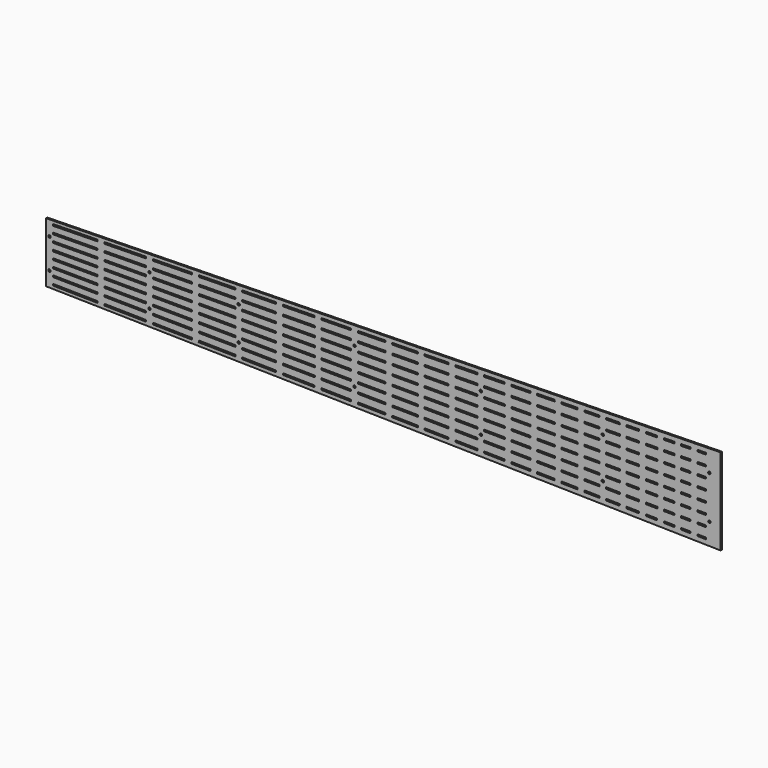
from build123d import *

# Parameters (mm, degrees)
F2_DEPTH = 1.524
F4_DEPTH = 1.525
F5_R     = 1.1303
F6_DEPTH = 985
F7_DEPTH = 1.525


# Not quite as in the source:
# - an extrude ends at something that could not be found from the text; its depth is read off the source's solid


with BuildPart() as f2:
    # F1 (on Front) → F2 (new body)
    with BuildSketch(Plane.XZ):
        Polygon((0, 56.388), (0, 0), (635, -12.446), (635, 68.834), align=None)
    extrude(amount=F2_DEPTH)

    # F0 (on Front) → F4 (cut, through all)
    with BuildSketch(Plane.XZ):
        Polygon((6.3619321188, 4.1792032166), (6.3490994724, 3.4173112799), (6.336266826, 2.6554193432), (48.4507071038, 1.946080269), (48.4635397502, 2.7079722057), (48.4763723966, 3.4698641423), align=None)
        Polygon((54.825471869, 3.3629254222), (54.8126392226, 2.6010334855), (54.7998065761, 1.8391415489), (94.1934291625, 1.175629566), (94.2062618089, 1.9375215027), (94.2190944553, 2.6994134394), align=None)
        Polygon((100.5681939277, 2.5924747193), (100.5553612812, 1.8305827826), (100.5425286348, 1.0686908459), (137.3698960072, 0.4484026382), (137.3827286536, 1.2102945749), (137.3955613, 1.9721865116), align=None)
        Polygon((143.7446607724, 1.8652477915), (143.731828126, 1.1033558548), (143.7189954796, 0.3414639181), (178.1148101324, -0.2378693263), (178.1276427788, 0.5240226104), (178.1404754253, 1.285914547), align=None)
        Polygon((184.4895748976, 1.1789758269), (184.4767422512, 0.4170838902), (184.4639096048, -0.3448080465), (216.5879148808, -0.8858769058), (216.6007475272, -0.1239849691), (216.6135801737, 0.6379069676), align=None)
        Polygon((222.962679646, 0.5309682475), (222.9498469996, -0.2309236892), (222.9370143532, -0.9928156259), (252.8936910333, -1.4973798837), (252.9065236798, -0.7354879471), (252.9193563262, 0.0264039896), align=None)
        Polygon((259.2684557986, -0.0805347305), (259.2556231521, -0.8424266672), (259.2427905057, -1.6043186039), (287.1625236967, -2.0745743538), (287.1753563432, -1.3126824171), (287.1881889896, -0.5507904804), align=None)
        Polygon((293.5372884619, -0.6577292005), (293.5244558155, -1.4196211372), (293.5116231691, -2.1815130739), (319.5075284272, -2.6193655361), (319.5203610736, -1.8574735994), (319.53319372, -1.0955816627), align=None)
        Polygon((325.8822931924, -1.2025203828), (325.869460546, -1.9644123195), (325.8566278996, -2.7263042562), (350.0375033933, -3.1335859326), (350.0503360397, -2.3716939959), (350.0631686861, -1.6098020592), align=None)
        Polygon((356.4122681585, -1.7167407793), (356.3994355121, -2.478632716), (356.3866028657, -3.2405246527), (378.8543389434, -3.6189516959), (378.8671715898, -2.8570597592), (378.8800042362, -2.0951678225), align=None)
        Polygon((385.2291037086, -2.2021065426), (385.2162710622, -2.9639984793), (385.2034384157, -3.725890416), (406.0530176055, -4.0770626292), (406.0658502519, -3.3151706925), (406.0786828983, -2.5532787558), align=None)
        Polygon((412.4277823707, -2.6602174759), (412.4149497243, -3.4221094126), (412.4021170779, -4.1840013493), (431.7259314752, -4.5094749048), (431.7387641216, -3.7475829681), (431.7515967681, -2.9856910314), align=None)
        Polygon((438.1006962404, -3.0926297515), (438.087863594, -3.8545216882), (438.0750309476, -4.6164136249), (455.9577013503, -4.917613802), (455.9705339967, -4.1557218653), (455.9833666431, -3.3938299286), align=None)
        Polygon((462.3324661155, -3.5007686487), (462.3196334691, -4.2626605854), (462.3068008227, -5.0245525221), (478.8294941184, -5.3028464253), (478.8423267648, -4.5409544886), (478.8551594113, -3.7790625519), align=None)
        Polygon((485.2042588836, -3.886001272), (485.1914262372, -4.6478932087), (485.1785935908, -5.4097851454), (500.417295802, -5.6664526173), (500.4301284485, -4.9045606807), (500.4429610949, -4.142668744), align=None)
        Polygon((506.7920605672, -4.2496074641), (506.7792279208, -5.0114994008), (506.7663952744, -5.7733913375), (520.7936385135, -6.0096540461), (520.8064711599, -5.2477621094), (520.8193038064, -4.4858701727), align=None)
        Polygon((527.1684032787, -4.5928088929), (527.1555706323, -5.3547008295), (527.1427379859, -6.1165927662), (540.0258735001, -6.3335851175), (540.0387061465, -5.5716931808), (540.0515387929, -4.8098012441), align=None)
        Polygon((546.4006382653, -4.9167399643), (546.3878056189, -5.6786319009), (546.3749729725, -6.4405238376), (558.1796250539, -6.6393511502), (558.1924577003, -5.8774592135), (558.2052903467, -5.1155672768), align=None)
        Polygon((564.5543898191, -5.2225059969), (564.5415571727, -5.9843979336), (564.5287245263, -6.7462898703), (575.3136096468, -6.9279411133), (575.3264422932, -6.1660491766), (575.3392749396, -5.40415724), align=None)
        Polygon((581.688374412, -5.5110959601), (581.6755417656, -6.2729878968), (581.6627091192, -7.0348798334), (591.4865437508, -7.2003439763), (591.4993763972, -6.4384520396), (591.5122090436, -5.6765601029), align=None)
        Polygon((597.861308516, -5.7834988231), (597.8484758696, -6.5453907597), (597.8356432232, -7.3072826964), (606.7510994951, -7.4574469027), (606.7639321415, -6.695554966), (606.7767647879, -5.9336630294), align=None)
        Polygon((613.1258642603, -6.0406017495), (613.1130316139, -6.8024936862), (613.1001989675, -7.5643856228), (621.1599490089, -7.7001370562), (621.1727816553, -6.9382451195), (621.1856143017, -6.1763531828), align=None)
        Polygon((6.3587067391, 11.2583100675), (6.3495405631, 10.4963651999), (6.3403743871, 9.7344203323), (48.4577404796, 9.227749565), (48.4669066556, 9.9896944326), (48.4760728316, 10.7516393002), align=None)
        Polygon((54.8256133947, 10.6752545001), (54.8164472187, 9.9133096325), (54.8072810427, 9.151364765), (94.2036404204, 8.6774276344), (94.2128065964, 9.4393725019), (94.2219727724, 10.2013173695), align=None)
        Polygon((100.5715133355, 10.1249325694), (100.5623471595, 9.3629877018), (100.5531809835, 8.6010428343), (137.383106862, 8.1579798288), (137.392273038, 8.9199246963), (137.401439214, 9.6818695639), align=None)
        Polygon((143.7509797771, 9.6054847638), (143.7418136011, 8.8435398963), (143.732647425, 8.0815950287), (178.1308516568, 7.6677855684), (178.1400178328, 8.429730436), (178.1491840088, 9.1916753035), align=None)
        Polygon((184.4987245719, 9.1152905035), (184.4895583959, 8.3533456359), (184.4803922199, 7.5914007683), (216.6066292456, 7.2049230116), (216.6157954216, 7.9668678792), (216.6249615976, 8.7288127468), align=None)
        Polygon((222.9745021607, 8.6524279467), (222.9653359847, 7.8904830791), (222.9561698087, 7.1285382116), (252.9149276677, 6.7681351702), (252.9240938437, 7.5300800378), (252.9332600197, 8.2920249054), align=None)
        Polygon((259.2828005828, 8.2156401053), (259.2736344068, 7.4536952377), (259.2644682308, 6.6917503702), (287.1861410882, 6.355853406), (287.1953072642, 7.1177982735), (287.2044734402, 7.8797431411), align=None)
        Polygon((293.5540140033, 7.803358341), (293.5448478273, 7.0414134734), (293.5356816513, 6.2794686059), (319.5333929218, 5.9667168472), (319.5425590978, 6.7286617147), (319.5517252738, 7.4906065823), align=None)
        Polygon((325.9012658369, 7.4142217822), (325.8920996609, 6.6522769147), (325.8829334849, 5.8903320471), (350.0654888955, 5.5994165639), (350.0746550715, 6.3613614315), (350.0838212475, 7.1233062991), align=None)
        Polygon((356.4333618106, 7.046921499), (356.4241956346, 6.2849766314), (356.4150294586, 5.5230317639), (378.8843264363, 5.252726733), (378.8934926124, 6.0146716006), (378.9026587884, 6.7766164682), align=None)
        Polygon((385.2521993515, 6.7002316681), (385.2430331754, 5.9382868005), (385.2338669994, 5.1763419329), (406.0848946711, 4.9255046378), (406.0940608471, 5.6874495054), (406.1032270231, 6.4493943729), align=None)
        Polygon((412.4527675862, 6.3730095728), (412.4436014102, 5.6110647053), (412.4344352342, 4.8491198377), (431.7595921141, 4.6166387266), (431.7687582901, 5.3785835942), (431.7779244661, 6.1405284618), align=None)
        Polygon((438.1274650292, 6.0641436617), (438.1182988532, 5.3021987941), (438.1091326771, 4.5402539266), (455.9930454418, 4.3251109429), (456.0022116179, 5.0870558105), (456.0113777939, 5.8490006781), align=None)
        Polygon((462.360918357, 5.772615878), (462.3517521809, 5.0106710104), (462.3425860049, 4.2487261429), (478.866427181, 4.0499447834), (478.875593357, 4.811889651), (478.884759533, 5.5738345186), align=None)
        Polygon((485.2343000961, 5.4974497185), (485.2251339201, 4.7355048509), (485.2159677441, 3.9735599833), (500.455728633, 3.7902260748), (500.4648948091, 4.5521709424), (500.4740609851, 5.31411581), align=None)
        Polygon((506.8236015482, 5.2377310099), (506.8144353721, 4.4757861423), (506.8052691961, 3.7138412747), (520.8334869493, 3.5450821971), (520.8426531253, 4.3070270647), (520.8518193013, 5.0689719323), align=None)
        Polygon((527.2013598644, 4.9925871322), (527.1921936884, 4.2306422646), (527.1830275124, 3.468697397), (540.0670580561, 3.3137028604), (540.0762242321, 4.075647728), (540.0853904081, 4.8375925956), align=None)
        Polygon((546.4349309712, 4.7612077955), (546.4257647952, 3.9992629279), (546.4165986192, 3.2373180603), (558.2220708047, 3.0952985514), (558.2312369807, 3.857243419), (558.2404031567, 4.6191882865), align=None)
        Polygon((564.5899437198, 4.5428034864), (564.5807775438, 3.7808586189), (564.5716113678, 3.0189137513), (575.3572457462, 2.8891628634), (575.3664119222, 3.651107731), (575.3755780982, 4.4130525985), align=None)
        Polygon((581.7251186613, 4.3366677985), (581.7159524853, 3.5747229309), (581.7067863093, 2.8127780633), (591.5313034317, 2.6945893898), (591.5404696077, 3.4565342574), (591.5496357837, 4.218479125), align=None)
        Polygon((597.8991763468, 4.1420943249), (597.8900101708, 3.3801494573), (597.8808439948, 2.6182045898), (606.7969196498, 2.5109444424), (606.8060858258, 3.27288931), (606.8152520018, 4.0348341775), align=None)
        Polygon((613.1647925649, 3.9584493775), (613.1556263889, 3.1965045099), (613.1464602129, 2.4345596423), (621.206770189, 2.3375943328), (621.215936365, 3.0995392003), (621.225102541, 3.8614840679), align=None)
        Polygon((6.3553343121, 18.3373992727), (6.3498346065, 17.5754191199), (6.3443349009, 16.8134389672), (48.4636514236, 16.5094365068), (48.4691511292, 17.2714166596), (48.4746508348, 18.0333968124), align=None)
        Polygon((54.8244854414, 17.9875659323), (54.8189857358, 17.2255857795), (54.8134860302, 16.4636056267), (94.2116698299, 16.1792433484), (94.2171695355, 16.9412235012), (94.2226692411, 17.7032036539), align=None)
        Polygon((100.5725038477, 17.6573727739), (100.5670041421, 16.8953926211), (100.5615044365, 16.1334124683), (137.3931358869, 15.867574665), (137.3986355925, 16.6295548178), (137.4041352981, 17.3915349706), align=None)
        Polygon((143.7539699047, 17.3457040905), (143.7484701991, 16.5837239378), (143.7429704935, 15.821743785), (178.1427676857, 15.5734581088), (178.1482673913, 16.3354382616), (178.1537670969, 17.0974184144), align=None)
        Polygon((184.5036017034, 17.0515875343), (184.4981019978, 16.2896073815), (184.4926022922, 15.5276272287), (216.6203270648, 15.2957405747), (216.6258267704, 16.0577207275), (216.631326476, 16.8197008803), align=None)
        Polygon((222.9811610826, 16.7738700003), (222.975661377, 16.0118898475), (222.9701616713, 15.2499096947), (252.9303069027, 15.0336678699), (252.9358066083, 15.7956480227), (252.9413063139, 16.5576281755), align=None)
        Polygon((259.2911409204, 16.5117972954), (259.2856412148, 15.7498171426), (259.2801415092, 14.9878369899), (287.2031074027, 14.7862988113), (287.2086071083, 15.5482789641), (287.2141068139, 16.3102591169), align=None)
        Polygon((293.5639414205, 16.2644282368), (293.5584417149, 15.5024480841), (293.5529420093, 14.7404679313), (319.5518572183, 14.5528168761), (319.5573569239, 15.3147970288), (319.5628566295, 16.0767771816), align=None)
        Polygon((325.9126912361, 16.0309463016), (325.9071915305, 15.2689661488), (325.9016918249, 14.506985996), (350.0853671153, 14.3324367061), (350.0908668209, 15.0944168589), (350.0963665265, 15.8563970117), align=None)
        Polygon((356.446201133, 15.8105661316), (356.4407014274, 15.0485859789), (356.4352017218, 14.2866058261), (378.9055392394, 14.1244228076), (378.911038945, 14.8864029604), (378.9165386506, 15.6483831131), align=None)
        Polygon((385.2663732571, 15.6025522331), (385.2608735515, 14.8405720803), (385.2553738459, 14.0785919275), (406.1073671163, 13.9280895504), (406.1128668219, 14.6900697032), (406.1183665275, 15.452049856), align=None)
        Polygon((412.468201134, 15.406218976), (412.4627014284, 14.6442388232), (412.4572017228, 13.8822586704), (431.7832535392, 13.7427700037), (431.7887532448, 14.5047501565), (431.7942529504, 15.2667303093), align=None)
        Polygon((438.144087557, 15.2208994293), (438.1385878514, 14.4589192765), (438.1330881458, 13.6969391237), (456.0178291038, 13.5678533335), (456.0233288095, 14.3298334863), (456.0288285151, 15.0918136391), align=None)
        Polygon((462.3786631216, 15.045982759), (462.373163416, 14.2840026063), (462.3676637104, 13.5220224535), (478.8922700957, 13.4027536378), (478.8977698013, 14.1647337906), (478.903269507, 14.9267139434), align=None)
        Polygon((485.2531041135, 14.8808830633), (485.2476044079, 14.1189029106), (485.2421047023, 13.3569227578), (500.4825713355, 13.2469224126), (500.4880710411, 14.0089025654), (500.4935707467, 14.7708827182), align=None)
        Polygon((506.8434053532, 14.7250518382), (506.8379056476, 13.9630716854), (506.832405942, 13.2010915326), (520.8612733336, 13.099836086), (520.8667730392, 13.8618162388), (520.8722727448, 14.6237963916), align=None)
        Polygon((527.2221073514, 14.5779655116), (527.2166076458, 13.8159853588), (527.2111079402, 13.054005206), (540.0957351357, 12.961008484), (540.1012348413, 13.7229886368), (540.1067345469, 14.4849687896), align=None)
        Polygon((546.4565691534, 14.4391379095), (546.4510694478, 13.6771577567), (546.4455697422, 12.915177604), (558.2515886321, 12.8299658986), (558.2570883377, 13.5919460514), (558.2625880433, 14.3539262042), align=None)
        Polygon((564.6124226499, 14.3080953241), (564.6069229443, 13.5461151713), (564.6014232387, 12.7841350185), (575.3875570934, 12.7062844858), (575.393056799, 13.4682646386), (575.3985565046, 14.2302447914), align=None)
        Polygon((581.7483911111, 14.1844139113), (581.7428914055, 13.4224337585), (581.7373916999, 12.6604536057), (591.5623637899, 12.5895404017), (591.5678634955, 13.3515205544), (591.5733632012, 14.1135007072), align=None)
        Polygon((597.9231978077, 14.0676698272), (597.9176981021, 13.3056896744), (597.9121983965, 12.5437095216), (606.8286869497, 12.4793534332), (606.8341866553, 13.241333586), (606.8396863609, 14.0033137388), align=None)
        Polygon((613.1895209674, 13.9574828587), (613.1840212618, 13.1955027059), (613.1785215562, 12.4335225531), (621.2392048005, 12.3753433674), (621.2447045061, 13.1373235202), (621.2502042117, 13.899303673), align=None)
        Polygon((6.3518148584, 25.4164708348), (6.3499816232, 24.65447304), (6.348148388, 23.8924752452), (48.4684400919, 23.7911410917), (48.4702733271, 24.5531388865), (48.4721065623, 25.3151366813), align=None)
        Polygon((54.8220881855, 25.2998597213), (54.8202549503, 24.5378619265), (54.8184217151, 23.7758641317), (94.2175176941, 23.6810767056), (94.2193509293, 24.4430745004), (94.2211841645, 25.2050722952), align=None)
        Polygon((100.5711657877, 25.1897953351), (100.5693325525, 24.4277975404), (100.5674993173, 23.6657997456), (137.3999835241, 23.5771871445), (137.4018167593, 24.3391849393), (137.4036499945, 25.101182734), align=None)
        Polygon((143.7536316177, 25.085905774), (143.7517983825, 24.3239079793), (143.7499651473, 23.5619101845), (178.150558792, 23.4791482924), (178.1523920272, 24.2411460872), (178.1542252624, 25.003143882), align=None)
        Polygon((184.5042068856, 24.987866922), (184.5023736504, 24.2258691272), (184.5005404152, 23.4638713324), (216.6290090354, 23.3865757811), (216.6308422706, 24.1485735758), (216.6326755058, 24.9105713706), align=None)
        Polygon((222.982657129, 24.8952944106), (222.9808238938, 24.1332966158), (222.9789906586, 23.371298821), (252.939829552, 23.2992182128), (252.9416627872, 24.0612160076), (252.9434960224, 24.8232138023), align=None)
        Polygon((259.2934776455, 24.8079368423), (259.2916444103, 24.0459390475), (259.2898111751, 23.2839412528), (287.2134235642, 23.2167618599), (287.2152567994, 23.9787596547), (287.2170900346, 24.7407574495), align=None)
        Polygon((293.5670716578, 24.7254804895), (293.5652384226, 23.9634826947), (293.5634051874, 23.2014848999), (319.5629223448, 23.1389345482), (319.56475558, 23.9009323429), (319.5665888152, 24.6629301377), align=None)
        Polygon((325.9165704384, 24.6476531777), (325.9147372032, 23.8856553829), (325.912903968, 23.1236575882), (350.0971391788, 23.0654744915), (350.098972414, 23.8274722863), (350.1008056493, 24.5894700811), align=None)
        Polygon((356.4507872724, 24.5741931211), (356.4489540372, 23.8121953263), (356.447120802, 23.0501975315), (378.9179785714, 22.9961365253), (378.9198118066, 23.7581343201), (378.9216450418, 24.5201321149), align=None)
        Polygon((385.2716266649, 24.5048551549), (385.2697934297, 23.7428573601), (385.2679601945, 22.9808595653), (406.1204362475, 22.9306921063), (406.1222694827, 23.6926899011), (406.1241027179, 24.4546876959), align=None)
        Polygon((412.4740843411, 24.4394107358), (412.4722511059, 23.6774129411), (412.4704178707, 22.9154151463), (431.7969171398, 22.8689189241), (431.798750375, 23.6309167188), (431.8005836102, 24.3929145136), align=None)
        Polygon((438.1505652334, 24.3776375536), (438.1487319982, 23.6156397588), (438.146898763, 22.853641964), (456.0320538033, 22.8106133673), (456.0338870385, 23.5726111621), (456.0357202738, 24.3346089569), align=None)
        Polygon((462.3857018969, 24.3193319969), (462.3838686617, 23.5573342021), (462.3820354265, 22.7953364073), (478.9070244032, 22.7555801354), (478.9088576384, 23.5175779302), (478.9106908736, 24.279575725), align=None)
        Polygon((485.2606724968, 24.264298765), (485.2588392616, 23.5023009702), (485.2570060264, 22.7403031754), (500.4978255195, 22.7036363937), (500.4996587547, 23.4656341885), (500.5014919899, 24.2276319833), align=None)
        Polygon((506.851473613, 24.2123550232), (506.8496403778, 23.4503572285), (506.8478071426, 22.6883594337), (520.8769993422, 22.6546076182), (520.8788325774, 23.4166054129), (520.8806658126, 24.1786032077), align=None)
        Polygon((527.2306474357, 24.1633262477), (527.2288142005, 23.4013284529), (527.2269809653, 22.6393306581), (540.1119064764, 22.6083317508), (540.1137397116, 23.3703295456), (540.1155729468, 24.1323273404), align=None)
        Polygon((546.4655545699, 24.1170503804), (546.4637213347, 23.3550525856), (546.4618880995, 22.5930547908), (558.2681803321, 22.564650889), (558.2700135673, 23.3266486838), (558.2718468025, 24.0886464786), align=None)
        Polygon((564.6218284257, 24.0733695186), (564.6199951905, 23.3113717238), (564.6181619553, 22.549373929), (575.4045455395, 22.5234237514), (575.4063787747, 23.2854215462), (575.4082120099, 24.047419341), align=None)
        Polygon((581.7581936331, 24.032142381), (581.7563603979, 23.2701445862), (581.7545271627, 22.5081467914), (591.5797267286, 22.4845090567), (591.5815599638, 23.2465068515), (591.583393199, 24.0085046463), align=None)
        Polygon((597.9333748221, 23.9932276862), (597.9315415869, 23.2312298915), (597.9297083517, 22.4692320967), (606.8464033468, 22.4477800672), (606.848236582, 23.209777862), (606.8500698172, 23.9717756568), align=None)
        Polygon((613.2000514404, 23.9564986968), (613.1982182052, 23.194500902), (613.19638497, 22.4325031072), (621.2572548418, 22.4131100453), (621.259088077, 23.1751078401), (621.2609213122, 23.9371056348), align=None)
        Polygon((216.6258267704, 40.3302792725), (216.6203270648, 41.0922594253), (184.4926022922, 40.8603727713), (184.4981019978, 40.0983926185), (184.5036017034, 39.3364124657), (216.631326476, 39.5682991197), align=None)
        Polygon((94.2062618089, 54.4504784973), (94.1934291625, 55.212370434), (54.7998065761, 54.5488584511), (54.8126392226, 53.7869665145), (54.825471869, 53.0250745778), (94.2190944553, 53.6885865606), align=None)
        Polygon((48.4635397502, 53.6800277943), (48.4507071038, 54.441919731), (6.336266826, 53.7325806568), (6.3490994724, 52.9706887201), (6.3619321188, 52.2087967834), (48.4763723966, 52.9181358577), align=None)
        Polygon((184.4987245719, 47.2727094965), (216.6249615976, 47.6591872532), (216.6157954216, 48.4211321208), (216.6066292456, 49.1830769884), (184.4803922199, 48.7965992317), (184.4895583959, 48.0346543641), align=None)
        Polygon((325.9012658369, 48.9737782178), (350.0838212475, 49.2646937009), (350.0746550715, 50.0266385685), (350.0654888955, 50.7885834361), (325.8829334849, 50.4976679529), (325.8920996609, 49.7357230853), align=None)
        Polygon((356.4150294586, 50.8649682361), (356.4241956346, 50.1030233686), (356.4333618106, 49.341078501), (378.9026587884, 49.6113835318), (378.8934926124, 50.3733283994), (378.8843264363, 51.135273267), align=None)
        Polygon((6.3443349009, 39.5745610328), (6.3498346065, 38.8125808801), (6.3553343121, 38.0506007273), (48.4746508348, 38.3546031876), (48.4691511292, 39.1165833404), (48.4636514236, 39.8785634932), align=None)
        Polygon((100.5425286348, 55.3193091541), (100.5553612812, 54.5574172174), (100.5681939277, 53.7955252807), (137.3955613, 54.4158134884), (137.3827286536, 55.1777054251), (137.3698960072, 55.9395973618), align=None)
        Polygon((325.9016918249, 41.881014004), (325.9071915305, 41.1190338512), (325.9126912361, 40.3570536984), (350.0963665265, 40.5316029883), (350.0908668209, 41.2935831411), (350.0853671153, 42.0555632939), align=None)
        Polygon((319.5425590978, 49.6593382853), (319.5333929218, 50.4212831528), (293.5356816513, 50.1085313941), (293.5448478273, 49.3465865266), (293.5540140033, 48.584641659), (319.5517252738, 48.8973934177), align=None)
        Polygon((540.0762242321, 52.312352272), (540.0670580561, 53.0742971396), (527.1830275124, 52.919302603), (527.1921936884, 52.1573577354), (527.2013598644, 51.3954128678), (540.0853904081, 51.5504074044), align=None)
        Polygon((54.8256133947, 45.7127454999), (94.2219727724, 46.1866826305), (94.2128065964, 46.9486274981), (94.2036404204, 47.7105723656), (54.8072810427, 47.236635235), (54.8164472187, 46.4746903675), align=None)
        Polygon((412.4572017228, 42.5057413296), (412.4627014284, 41.7437611768), (412.468201134, 40.981781024), (431.7942529504, 41.1212696907), (431.7887532448, 41.8832498435), (431.7832535392, 42.6452299963), align=None)
        Polygon((520.8426531253, 52.0809729353), (520.8334869493, 52.8429178029), (506.8052691961, 52.6741587253), (506.8144353721, 51.9122138577), (506.8236015482, 51.1502689901), (520.8518193013, 51.3190280677), align=None)
        Polygon((259.2828005828, 48.1723598947), (287.2044734402, 48.5082568589), (287.1953072642, 49.2702017265), (287.1861410882, 50.032146594), (259.2644682308, 49.6962496298), (259.2736344068, 48.9343047623), align=None)
        Polygon((546.4165986192, 53.1506819397), (546.4257647952, 52.3887370721), (546.4349309712, 51.6267922045), (558.2404031567, 51.7688117135), (558.2312369807, 52.530756581), (558.2220708047, 53.2927014486), align=None)
        Polygon((606.8060858258, 53.11511069), (606.7969196498, 53.8770555576), (597.8808439948, 53.7697954102), (597.8900101708, 53.0078505427), (597.8991763468, 52.2459056751), (606.8152520018, 52.3531658225), align=None)
        Polygon((613.1785215562, 43.9544774469), (613.1840212618, 43.1924972941), (613.1895209674, 42.4305171413), (621.2502042117, 42.488696327), (621.2447045061, 43.2506764798), (621.2392048005, 44.0126566326), align=None)
        Polygon((184.5005404152, 32.9241286676), (184.5023736504, 32.1621308728), (184.5042068856, 31.400133078), (216.6326755058, 31.4774286294), (216.6308422706, 32.2394264242), (216.6290090354, 33.0014242189), align=None)
        Polygon((462.3786631216, 41.342017241), (478.903269507, 41.4612860566), (478.8977698013, 42.2232662094), (478.8922700957, 42.9852463622), (462.3676637104, 42.8659775465), (462.373163416, 42.1039973937), align=None)
        Polygon((178.1400178328, 47.958269564), (178.1308516568, 48.7202144316), (143.732647425, 48.3064049713), (143.7418136011, 47.5444601037), (143.7509797771, 46.7825152362), (178.1491840088, 47.1963246965), align=None)
        Polygon((6.3587067391, 45.1296899325), (48.4760728316, 45.6363606998), (48.4669066556, 46.3983055674), (48.4577404796, 47.160250435), (6.3403743871, 46.6535796677), (6.3495405631, 45.8916348001), align=None)
        Polygon((178.1523920272, 32.1468539128), (178.150558792, 32.9088517076), (143.7499651473, 32.8260898155), (143.7517983825, 32.0640920207), (143.7536316177, 31.302094226), (178.1542252624, 31.384856118), align=None)
        Polygon((478.875593357, 51.576110349), (478.866427181, 52.3380552166), (462.3425860049, 52.1392738571), (462.3517521809, 51.3773289896), (462.360918357, 50.615384122), (478.884759533, 50.8141654814), align=None)
        Polygon((100.5725038477, 38.7306272261), (137.4041352981, 38.9964650294), (137.3986355925, 39.7584451822), (137.3931358869, 40.520425335), (100.5615044365, 40.2545875317), (100.5670041421, 39.4926073789), align=None)
        Polygon((293.5529420093, 41.6475320687), (293.5584417149, 40.8855519159), (293.5639414205, 40.1235717632), (319.5628566295, 40.3112228184), (319.5573569239, 41.0732029712), (319.5518572183, 41.8351831239), align=None)
        Polygon((259.2801415092, 41.4001630101), (259.2856412148, 40.6381828574), (259.2911409204, 39.8762027046), (287.2141068139, 40.0777408831), (287.2086071083, 40.8397210359), (287.2031074027, 41.6017011887), align=None)
        Polygon((222.9701616713, 41.1380903053), (222.975661377, 40.3761101525), (222.9811610826, 39.6141299997), (252.9413063139, 39.8303718245), (252.9358066083, 40.5923519773), (252.9303069027, 41.3543321301), align=None)
        Polygon((606.8341866553, 43.146666414), (606.8286869497, 43.9086465668), (597.9121983965, 43.8442904784), (597.9176981021, 43.0823103256), (597.9231978077, 42.3203301728), (606.8396863609, 42.3846862612), align=None)
        Polygon((54.8134860302, 39.9243943733), (54.8189857358, 39.1624142205), (54.8244854414, 38.4004340677), (94.2226692411, 38.6847963461), (94.2171695355, 39.4467764988), (94.2116698299, 40.2087566516), align=None)
        Polygon((581.6627091192, 63.4228798334), (581.6755417656, 62.6609878968), (581.688374412, 61.8990959601), (591.5122090436, 62.0645601029), (591.4993763972, 62.8264520396), (591.4865437508, 63.5883439763), align=None)
        Polygon((184.4895748976, 55.2090241731), (216.6135801737, 55.7500930324), (216.6007475272, 56.5119849691), (216.5879148808, 57.2738769058), (184.4639096048, 56.7328080465), (184.4767422512, 55.9709161098), align=None)
        Polygon((54.8220881855, 31.0881402787), (94.2211841645, 31.1829277048), (94.2193509293, 31.9449254996), (94.2175176941, 32.7069232944), (54.8184217151, 32.6121358683), (54.8202549503, 31.8501380735), align=None)
        Polygon((143.7429704935, 40.566256215), (143.7484701991, 39.8042760622), (143.7539699047, 39.0422959095), (178.1537670969, 39.2905815856), (178.1482673913, 40.0525617384), (178.1427676857, 40.8145418912), align=None)
        Polygon((575.393056799, 42.9197353614), (575.3875570934, 43.6817155142), (564.6014232387, 43.6038649815), (564.6069229443, 42.8418848287), (564.6124226499, 42.0799046759), (575.3985565046, 42.1577552086), align=None)
        Polygon((500.4648948091, 51.8358290576), (500.455728633, 52.5977739252), (485.2159677441, 52.4144400167), (485.2251339201, 51.6524951491), (485.2343000961, 50.8905502815), (500.4740609851, 51.07388419), align=None)
        Polygon((438.1091326771, 51.8477460734), (438.1182988532, 51.0858012059), (438.1274650292, 50.3238563383), (456.0113777939, 50.5389993219), (456.0022116179, 51.3009441895), (455.9930454418, 52.0628890571), align=None)
        Polygon((412.4527675862, 50.0149904272), (431.7779244661, 50.2474715382), (431.7687582901, 51.0094164058), (431.7595921141, 51.7713612734), (412.4344352342, 51.5388801623), (412.4436014102, 50.7769352947), align=None)
        Polygon((575.3264422932, 62.5540491766), (575.3136096468, 63.3159411133), (564.5287245263, 63.1342898703), (564.5415571727, 62.3723979336), (564.5543898191, 61.6105059969), (575.3392749396, 61.79215724), align=None)
        Polygon((6.3518148584, 30.9715291652), (48.4721065623, 31.0728633187), (48.4702733271, 31.8348611135), (48.4684400919, 32.5968589083), (6.348148388, 32.4955247548), (6.3499816232, 31.73352696), align=None)
        Polygon((456.0233288095, 42.0581665137), (456.0178291038, 42.8201466665), (438.1330881458, 42.6910608763), (438.1385878514, 41.9290807235), (438.144087557, 41.1671005707), (456.0288285151, 41.2961863609), align=None)
        Polygon((137.4018167593, 32.0488150607), (137.3999835241, 32.8108128555), (100.5674993173, 32.7222002544), (100.5693325525, 31.9602024596), (100.5711657877, 31.1982046649), (137.4036499945, 31.286817266), align=None)
        Polygon((385.2034384157, 60.113890416), (385.2162710622, 59.3519984793), (385.2291037086, 58.5901065426), (406.0786828983, 58.9412787558), (406.0658502519, 59.7031706925), (406.0530176055, 60.4650626292), align=None)
        Polygon((293.5116231691, 58.5695130739), (293.5244558155, 57.8076211372), (293.5372884619, 57.0457292005), (319.53319372, 57.4835816627), (319.5203610736, 58.2454735994), (319.5075284272, 59.0073655361), align=None)
        Polygon((385.2338669994, 51.2116580671), (385.2430331754, 50.4497131995), (385.2521993515, 49.6877683319), (406.1032270231, 49.9386056271), (406.0940608471, 50.7005504946), (406.0848946711, 51.4624953622), align=None)
        Polygon((100.5531809835, 47.7869571657), (100.5623471595, 47.0250122982), (100.5715133355, 46.2630674306), (137.401439214, 46.7061304361), (137.392273038, 47.4680753037), (137.383106862, 48.2300201712), align=None)
        Polygon((613.1464602129, 53.9534403577), (613.1556263889, 53.1914954901), (613.1647925649, 52.4295506225), (621.225102541, 52.5265159321), (621.215936365, 53.2884607997), (621.206770189, 54.0504056672), align=None)
        Polygon((606.7639321415, 63.083554966), (606.7510994951, 63.8454469027), (597.8356432232, 63.6952826964), (597.8484758696, 62.9333907597), (597.861308516, 62.1714988231), (606.7767647879, 62.3216630294), align=None)
        Polygon((520.8064711599, 61.6357621094), (520.7936385135, 62.3976540461), (506.7663952744, 62.1613913375), (506.7792279208, 61.3994994008), (506.7920605672, 60.6376074641), (520.8193038064, 60.8738701727), align=None)
        Polygon((527.2111079402, 43.333994794), (527.2166076458, 42.5720146412), (527.2221073514, 41.8100344884), (540.1067345469, 41.9030312104), (540.1012348413, 42.6650113632), (540.0957351357, 43.426991516), align=None)
        Polygon((581.7067863093, 53.5752219367), (581.7159524853, 52.8132770691), (581.7251186613, 52.0513322015), (591.5496357837, 52.169520875), (591.5404696077, 52.9314657426), (591.5313034317, 53.6934106102), align=None)
        Polygon((575.3664119222, 52.736892269), (575.3572457462, 53.4988371366), (564.5716113678, 53.3690862487), (564.5807775438, 52.6071413811), (564.5899437198, 51.8451965136), (575.3755780982, 51.9749474015), align=None)
        Polygon((520.8667730392, 42.5261837612), (520.8612733336, 43.288163914), (506.832405942, 43.1869084674), (506.8379056476, 42.4249283146), (506.8434053532, 41.6629481618), (520.8722727448, 41.7642036084), align=None)
        Polygon((438.0750309476, 61.0044136249), (438.087863594, 60.2425216882), (438.1006962404, 59.4806297515), (455.9833666431, 59.7818299286), (455.9705339967, 60.5437218653), (455.9577013503, 61.305613802), align=None)
        Polygon((385.2663732571, 40.7854477669), (406.1183665275, 40.935950144), (406.1128668219, 41.6979302968), (406.1073671163, 42.4599104496), (385.2553738459, 42.3094080725), (385.2608735515, 41.5474279197), align=None)
        Polygon((178.1276427788, 55.8639773896), (178.1148101324, 56.6258693263), (143.7189954796, 56.0465360819), (143.731828126, 55.2846441452), (143.7446607724, 54.5227522085), (178.1404754252, 55.102085453), align=None)
        Polygon((356.4122681585, 58.1047407793), (378.8800042362, 58.4831678225), (378.8671715898, 59.2450597592), (378.8543389434, 60.0069516959), (356.3866028657, 59.6285246527), (356.3994355121, 58.866632716), align=None)
        Polygon((293.5634051874, 33.1865151001), (293.5652384226, 32.4245173053), (293.5670716578, 31.6625195105), (319.5665888152, 31.7250698623), (319.56475558, 32.4870676571), (319.5629223448, 33.2490654518), align=None)
        Polygon((485.2531041135, 41.5071169367), (500.4935707467, 41.6171172818), (500.4880710411, 42.3790974346), (500.4825713355, 43.1410775874), (485.2421047023, 43.0310772422), (485.2476044079, 42.2690970894), align=None)
        Polygon((222.9561698087, 49.2594617884), (222.9653359847, 48.4975169209), (222.9745021607, 47.7355720533), (252.9332600197, 48.0959750946), (252.9240938437, 48.8579199622), (252.9149276677, 49.6198648298), align=None)
        Polygon((259.2427905057, 57.9923186039), (259.2556231521, 57.2304266672), (259.2684557986, 56.4685347305), (287.1881889896, 56.9387904804), (287.1753563432, 57.7006824171), (287.1625236967, 58.4625743538), align=None)
        Polygon((356.4352017218, 42.1013941739), (356.4407014274, 41.3394140211), (356.446201133, 40.5774338684), (378.9165386506, 40.7396168869), (378.911038945, 41.5015970396), (378.9055392394, 42.2635771924), align=None)
        Polygon((485.2042588836, 60.274001272), (500.4429610949, 60.530668744), (500.4301284485, 61.2925606807), (500.417295802, 62.0544526173), (485.1785935908, 61.7977851454), (485.1914262372, 61.0358932087), align=None)
        Polygon((325.8566278996, 59.1143042562), (325.869460546, 58.3524123195), (325.8822931924, 57.5905203828), (350.0631686861, 57.9978020592), (350.0503360397, 58.7596939959), (350.0375033933, 59.5215859326), align=None)
        Polygon((581.7373916999, 43.7275463943), (581.7428914055, 42.9655662415), (581.7483911111, 42.2035860887), (591.5733632012, 42.2744992928), (591.5678634955, 43.0364794456), (591.5623637899, 43.7984595983), align=None)
        Polygon((613.1001989675, 63.9523856228), (613.1130316139, 63.1904936862), (613.1258642603, 62.4286017495), (621.1856143017, 62.5643531828), (621.1727816553, 63.3262451195), (621.1599490089, 64.0881370562), align=None)
        Polygon((558.2570883377, 42.7960539486), (558.2515886321, 43.5580341014), (546.4455697422, 43.472822396), (546.4510694478, 42.7108422433), (546.4565691534, 41.9488620905), (558.2625880433, 42.0340737958), align=None)
        Polygon((462.3324661155, 59.8887686487), (478.8551594113, 60.1670625519), (478.8423267648, 60.9289544886), (478.8294941184, 61.6908464253), (462.3068008227, 61.4125525221), (462.3196334691, 60.6506605854), align=None)
        Polygon((527.1427379859, 62.5045927662), (527.1555706323, 61.7427008295), (527.1684032787, 60.9808088929), (540.0515387929, 61.1978012441), (540.0387061465, 61.9596931808), (540.0258735001, 62.7215851175), align=None)
        Polygon((431.7387641216, 60.1355829681), (431.7259314752, 60.8974749048), (412.4021170779, 60.5720013493), (412.4149497243, 59.8101094126), (412.4277823707, 59.0482174759), (431.7515967681, 59.3736910314), align=None)
        Polygon((546.3749729725, 62.8285238376), (546.3878056189, 62.0666319009), (546.4006382653, 61.3047399643), (558.2052903467, 61.5035672768), (558.1924577003, 62.2654592135), (558.1796250539, 63.0273511502), align=None)
        Polygon((222.9789906586, 33.016701179), (222.9808238938, 32.2547033842), (222.982657129, 31.4927055894), (252.9434960224, 31.5647861977), (252.9416627872, 32.3267839924), (252.939829552, 33.0887817872), align=None)
        Polygon((259.2934776455, 31.5800631577), (287.2170900346, 31.6472425505), (287.2152567994, 32.4092403453), (287.2134235642, 33.1712381401), (259.2898111751, 33.1040587472), (259.2916444103, 32.3420609525), align=None)
        Polygon((252.9065236798, 57.1234879471), (252.8936910333, 57.8853798837), (222.9370143532, 57.3808156259), (222.9498469996, 56.6189236892), (222.962679646, 55.8570317525), (252.9193563262, 56.3615960104), align=None)
        Polygon((406.1222694827, 32.6953100989), (406.1204362475, 33.4573078937), (385.2679601945, 33.4071404347), (385.2697934297, 32.6451426399), (385.2716266649, 31.8831448451), (406.1241027179, 31.9333123041), align=None)
        Polygon((325.912903968, 33.2643424118), (325.9147372032, 32.5023446171), (325.9165704384, 31.7403468223), (350.1008056493, 31.7985299189), (350.098972414, 32.5605277137), (350.0971391788, 33.3225255085), align=None)
        Polygon((356.447120802, 33.3378024685), (356.4489540372, 32.5758046737), (356.4507872724, 31.8138068789), (378.9216450418, 31.8678678851), (378.9198118066, 32.6298656799), (378.9179785714, 33.3918634747), align=None)
        Polygon((412.4704178707, 33.4725848537), (412.4722511059, 32.7105870589), (412.4740843411, 31.9485892642), (431.8005836102, 31.9950854864), (431.798750375, 32.7570832812), (431.7969171398, 33.5190810759), align=None)
        Polygon((478.9070244032, 33.6324198646), (462.3820354265, 33.5926635927), (462.3838686617, 32.8306657979), (462.3857018969, 32.0686680031), (478.9106908736, 32.108424275), (478.9088576384, 32.8704220698), align=None)
        Polygon((520.8769993422, 33.7333923818), (506.8478071426, 33.6996405663), (506.8496403778, 32.9376427715), (506.851473613, 32.1756449768), (520.8806658126, 32.2093967923), (520.8788325774, 32.9713945871), align=None)
        Polygon((485.2588392616, 32.8856990298), (485.2606724968, 32.123701235), (500.5014919899, 32.1603680167), (500.4996587547, 32.9223658115), (500.4978255195, 33.6843636063), (485.2570060264, 33.6476968246), align=None)
        Polygon((438.146898763, 33.534358036), (438.1487319982, 32.7723602412), (438.1505652334, 32.0103624464), (456.0357202738, 32.0533910431), (456.0338870385, 32.8153888379), (456.0320538033, 33.5773866327), align=None)
        Polygon((558.2681803321, 33.823349111), (546.4618880995, 33.7949452092), (546.4637213347, 33.0329474144), (546.4655545699, 32.2709496196), (558.2718468025, 32.2993535214), (558.2700135673, 33.0613513162), align=None)
        Polygon((540.1119064764, 33.7796682492), (527.2269809653, 33.7486693419), (527.2288142005, 32.9866715471), (527.2306474357, 32.2246737523), (540.1155729468, 32.2556726596), (540.1137397116, 33.0176704544), align=None)
        Polygon((613.2000514404, 32.4315013032), (621.2609213122, 32.4508943652), (621.259088077, 33.2128921599), (621.2572548418, 33.9748899547), (613.19638497, 33.9554968928), (613.1982182052, 33.193499098), align=None)
        Polygon((606.848236582, 33.178222138), (606.8464033468, 33.9402199328), (597.9297083517, 33.9187679033), (597.9315415869, 33.1567701085), (597.9333748221, 32.3947723138), (606.8500698172, 32.4162243432), align=None)
        Polygon((564.6181619553, 33.838626071), (564.6199951905, 33.0766282762), (564.6218284257, 32.3146304814), (575.4082120099, 32.340580659), (575.4063787747, 33.1025784538), (575.4045455395, 33.8645762486), align=None)
        Polygon((581.7545271627, 33.8798532086), (581.7563603979, 33.1178554138), (581.7581936331, 32.355857619), (591.583393199, 32.3794953537), (591.5815599638, 33.1414931485), (591.5797267286, 33.9034909433), align=None)
    extrude(amount=F4_DEPTH, mode=Mode.SUBTRACT)

    # F5 (on face) → F6 (cut, through all)
    with BuildSketch(Plane.XZ.offset(1.524)):
        with Locations((97.3946236, 13.1425326887)):
            Circle(F5_R)
        with Locations((3.175, 14.065885)):
            Circle(F5_R)
        with Locations((181.3279076, 12.3199865055)):
            Circle(F5_R)
        with Locations((290.391088, 11.2511673376)):
            Circle(F5_R)
        with Locations((409.2984448, 10.085875241)):
            Circle(F5_R)
        with Locations((524.05534, 8.961257668)):
            Circle(F5_R)
        with Locations((624.435886, 7.9775283172)):
            Circle(F5_R)
        with Locations((97.3946236, 43.2454673113)):
            Circle(F5_R)
        with Locations((3.175, 42.322115)):
            Circle(F5_R)
        with Locations((181.3279076, 44.0680134945)):
            Circle(F5_R)
        with Locations((290.391088, 45.1368326624)):
            Circle(F5_R)
        with Locations((409.2984448, 46.302124759)):
            Circle(F5_R)
        with Locations((524.05534, 47.426742332)):
            Circle(F5_R)
        with Locations((624.435886, 48.4104716828)):
            Circle(F5_R)
    extrude(amount=F6_DEPTH, mode=Mode.SUBTRACT)

    # F5 (on face) → F7 (cut, through all)
    with BuildSketch(Plane.XZ.offset(1.524)):
        with Locations((97.3946236, 13.1425326887)):
            Circle(F5_R)
        with Locations((3.175, 14.065885)):
            Circle(F5_R)
        with Locations((181.3279076, 12.3199865055)):
            Circle(F5_R)
        with Locations((290.391088, 11.2511673376)):
            Circle(F5_R)
        with Locations((409.2984448, 10.085875241)):
            Circle(F5_R)
        with Locations((524.05534, 8.961257668)):
            Circle(F5_R)
        with Locations((624.435886, 7.9775283172)):
            Circle(F5_R)
        with Locations((97.3946236, 43.2454673113)):
            Circle(F5_R)
        with Locations((3.175, 42.322115)):
            Circle(F5_R)
        with Locations((181.3279076, 44.0680134945)):
            Circle(F5_R)
        with Locations((290.391088, 45.1368326624)):
            Circle(F5_R)
        with Locations((409.2984448, 46.302124759)):
            Circle(F5_R)
        with Locations((524.05534, 47.426742332)):
            Circle(F5_R)
        with Locations((624.435886, 48.4104716828)):
            Circle(F5_R)
    extrude(amount=-F7_DEPTH, mode=Mode.SUBTRACT)


solid = f2.part
